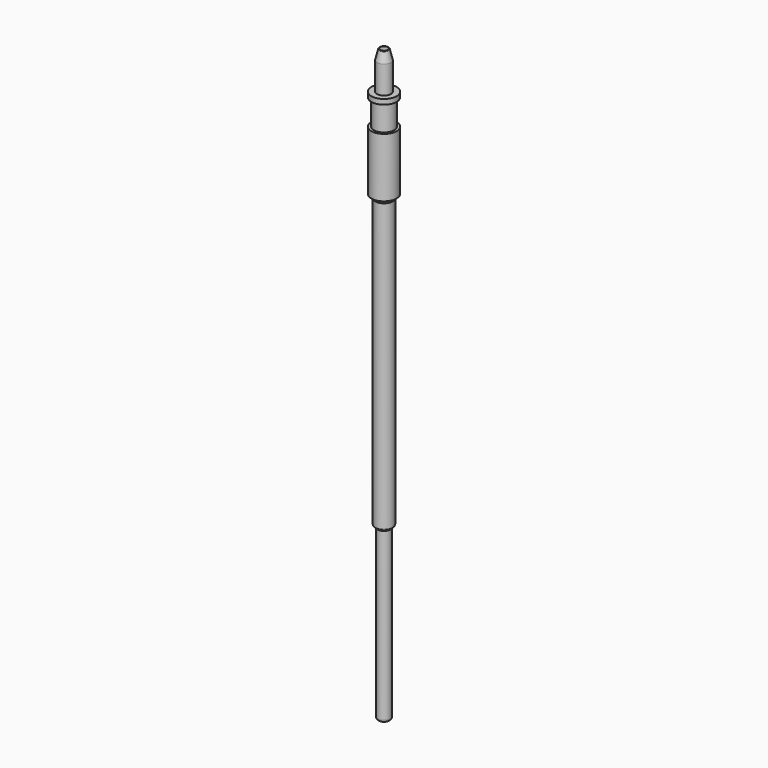
from build123d import *

# Parameters (mm, degrees)
F3_R        = 1.5
F4_DEPTH    = 235.059312583
F5_S5_R     = 3.5
F5_T6_DEPTH = 9
F6_SIZE2    = 4
F6_SIZE     = 1
F7_R        = 0.2
F8_R        = 0.5
F9_R        = 0.99999


# Not quite as in the source:
# - a fillet or chamfer that OpenCascade refuses, or shapes differently, is made with other operations: its cross-section is extruded or revolved along the edge and cut away or added
# - a fillet or chamfer is up to 0.001 mm smaller than in the source, because OpenCascade refuses the exact size


with BuildPart() as f1:
    # F0 (on Front) → F1 (revolve)
    with BuildSketch(Plane.XZ):
        Polygon((-1.5, -204.558312583), (-1.5, 29.441687417), (-2.75, 28.441687417), (-2.75, 14.441687417), (-5, 14.441687417), (-5, 12.441687417), (-4, 12.441687417), (-4, 2.241687417), (-5, 2.241687417), (-5, -22.258312583), (-3.5, -23.258312583), (-3.5, -136.558312583), (-2.5, -137.558312583), (-2.5, -204.558312583), align=None)
        Polygon((-5, -23.258312583), (-3.5, -23.258312583), (-5, -22.258312583), align=None)
        Polygon((-2.75, 28.441687417), (-1.5, 29.441687417), (-2.75, 29.441687417), align=None)
    revolve(axis=Axis((0, 0, -86.958312583), (0, 0, -1)))

    # F3 (on offset) → F4 (cut, through all)
    with BuildSketch(Plane.XY.offset(30.5)):
        Circle(F3_R)
    extrude(amount=-F4_DEPTH, mode=Mode.SUBTRACT)

    # F5: chamfer of 2 on 1 edges, made by hand


with BuildPart() as f5_tool2:
    # F5_s3 → F5_t4 (revolve)
    with BuildSketch(Plane.XZ):
        Polygon((-5, -21.258312583), (-3, -23.258312583), (-5, -23.258312583), align=None)
    revolve(axis=Axis((0, 0, -23.258312583), (0, 0, -1)))

    # F5_s5 → F5_t6 (cut, symmetric)
    with BuildSketch(Plane.XY.offset(-22.3)):
        Circle(F5_S5_R)
    extrude(amount=F5_T6_DEPTH, both=True, mode=Mode.SUBTRACT)


with BuildPart() as f1_1:
    add(f1.part)

    # F5_t1: cut F5_tool2
    add(f5_tool2.part, mode=Mode.SUBTRACT)

    # F6
    f6_edges = [f1_1.edges().sort_by_distance(p)[0] for p in [
        (2.75, 0, 29.441687),
    ]]
    chamfer(f6_edges, length=F6_SIZE, length2=F6_SIZE2)

    # F7
    f7_edges = [f1_1.edges().sort_by_distance(p)[0] for p in [
        (1.75, 0, 29.441687),
    ]]
    fillet(f7_edges, radius=F7_R)

    # F8
    f8_edges = [f1_1.edges().sort_by_distance(p)[0] for p in [
        (3.5, 0, -136.558313),
    ]]
    fillet(f8_edges, radius=F8_R)

    # F9 (radius 1 in the source; OpenCascade refuses exactly that, so slightly less here)
    f9_edges = [f1_1.edges().sort_by_distance(p)[0] for p in [
        (2.5, 0, -204.558313),
    ]]
    fillet(f9_edges, radius=F9_R)


solid = f1_1.part
